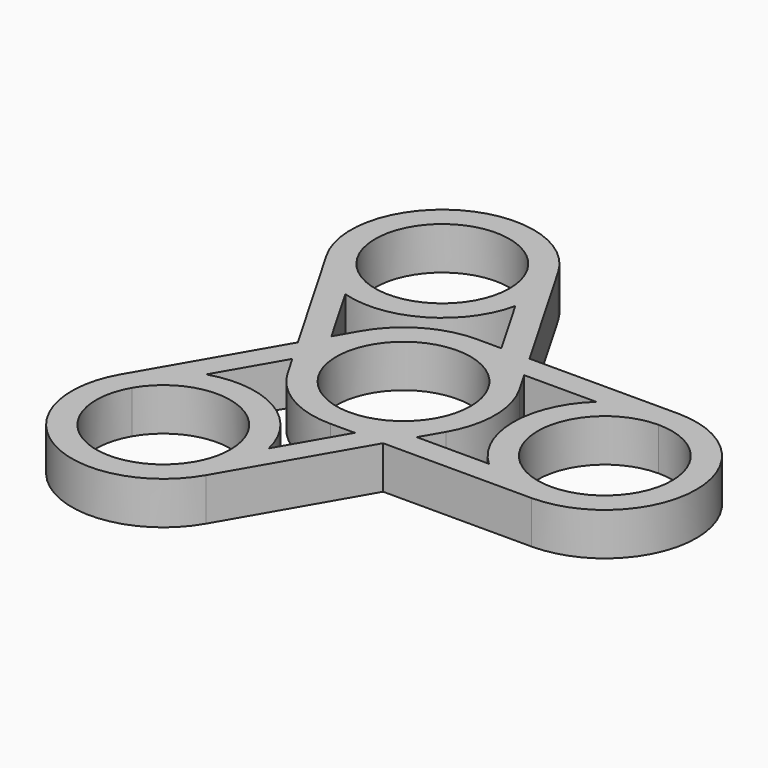
from build123d import *

# Parameters (mm, degrees)
F0_R     = 11
F1_DEPTH = 7


# Not quite as in the source:
# - a feature names something its author has since deleted; it is built from what else it names


with BuildPart() as f1:
    # F0 (on Top) → F1 (new body)
    with BuildSketch(Plane.XY):
        with BuildLine():
            Line((-15.0111069989, -4), (-12.9903810568, -7.5))
            ThreePointArc((-12.9903810568, -7.5), (-7.5, -12.9903810568), (0, -15))
            Line((0, -15), (4.0414518843, -15))
            Line((4.0414518843, -15), (-1.8747010448, -25.2470774586))
            ThreePointArc((-1.8747010448, -25.2470774586), (-1.5939696041, -26.9024559592), (-1.5, -28.5788383249))
            ThreePointArc((-1.5, -28.5788383249), (-2.0111126057, -32.4611240014), (-3.5096189432, -36.0788383249))
            Line((-3.5096189432, -36.0788383249), (8.6602540378, -15))
            Line((8.6602540378, -15), (33, -15))
            ThreePointArc((33, -15), (27.5227744249, -13.9642400438), (22.8019609728, -11))
            Line((22.8019609728, -11), (10.9696551146, -11))
            Line((10.9696551146, -11), (12.9903810568, -7.5))
            ThreePointArc((12.9903810568, -7.5), (15, 0), (12.9903810568, 7.5))
            Line((12.9903810568, 7.5), (10.9696551146, 11))
            Line((10.9696551146, 11), (22.8019609728, 11))
            ThreePointArc((22.8019609728, 11), (27.5227744249, 13.9642400438), (33, 15))
            Line((33, 15), (8.6602540378, 15))
            Line((8.6602540378, 15), (-3.5096189432, 36.0788383249))
            ThreePointArc((-3.5096189432, 36.0788383249), (-2.0111126057, 32.4611240014), (-1.5, 28.5788383249))
            ThreePointArc((-1.5, 28.5788383249), (-1.5939696041, 26.9024559592), (-1.8747010448, 25.2470774586))
            Line((-1.8747010448, 25.2470774586), (4.0414518843, 15))
            Line((4.0414518843, 15), (0, 15))
            ThreePointArc((0, 15), (-7.5, 12.9903810568), (-12.9903810568, 7.5))
            Line((-12.9903810568, 7.5), (-15.0111069989, 4))
            Line((-15.0111069989, 4), (-20.927259928, 14.2470774586))
            ThreePointArc((-20.927259928, 14.2470774586), (-25.8547738349, 16.8533018127), (-29.4903810568, 21.0788383249))
            Line((-29.4903810568, 21.0788383249), (-17.3205080757, 0))
            Line((-17.3205080757, 0), (-29.4903810568, -21.0788383249))
            ThreePointArc((-29.4903810568, -21.0788383249), (-25.8547738349, -16.8533018127), (-20.927259928, -14.2470774586))
            Line((-20.927259928, -14.2470774586), (-15.0111069989, -4))
        make_face()
        Circle(F0_R, mode=Mode.SUBTRACT)
        with BuildLine():
            Line((-26.0262794416, -23.0788383249), (-20.927259928, -14.2470774586))
            ThreePointArc((-20.927259928, -14.2470774586), (-25.8547738349, -16.8533018127), (-29.4903810568, -21.0788383249))
            ThreePointArc((-29.4903810568, -21.0788383249), (-24, -41.5692193817), (-3.5096189432, -36.0788383249))
            ThreePointArc((-3.5096189432, -36.0788383249), (-2.0111126057, -32.4611240014), (-1.5, -28.5788383249))
            ThreePointArc((-1.5, -28.5788383249), (-1.5939696041, -26.9024559592), (-1.8747010448, -25.2470774586))
            Line((-1.8747010448, -25.2470774586), (-6.9737205584, -34.0788383249))
            ThreePointArc((-6.9737205584, -34.0788383249), (-22, -38.1051177665), (-26.0262794416, -23.0788383249))
        make_face()
        with BuildLine():
            ThreePointArc((-3.5096189432, 36.0788383249), (-24, 41.5692193817), (-29.4903810568, 21.0788383249))
            ThreePointArc((-29.4903810568, 21.0788383249), (-25.8547738349, 16.8533018127), (-20.927259928, 14.2470774586))
            Line((-20.927259928, 14.2470774586), (-26.0262794416, 23.0788383249))
            ThreePointArc((-26.0262794416, 23.0788383249), (-22, 38.1051177665), (-6.9737205584, 34.0788383249))
            Line((-6.9737205584, 34.0788383249), (-1.8747010448, 25.2470774586))
            ThreePointArc((-1.8747010448, 25.2470774586), (-1.5939696041, 26.9024559592), (-1.5, 28.5788383249))
            ThreePointArc((-1.5, 28.5788383249), (-2.0111126057, 32.4611240014), (-3.5096189432, 36.0788383249))
        make_face()
        with BuildLine():
            ThreePointArc((22.8019609728, -11), (27.5227744249, -13.9642400438), (33, -15))
            ThreePointArc((33, -15), (43.6066017178, -10.6066017178), (48, 0))
            ThreePointArc((48, 0), (43.6066017178, 10.6066017178), (33, 15))
            ThreePointArc((33, 15), (27.5227744249, 13.9642400438), (22.8019609728, 11))
            Line((22.8019609728, 11), (33, 11))
            ThreePointArc((33, 11), (40.7781745931, 7.7781745931), (44, 0))
            ThreePointArc((44, 0), (40.7781745931, -7.7781745931), (33, -11))
            Line((33, -11), (22.8019609728, -11))
        make_face()
        with BuildLine():
            ThreePointArc((22.8019609728, 11), (18, 0), (22.8019609728, -11))
            Line((22.8019609728, -11), (33, -11))
            ThreePointArc((33, -11), (22, 0), (33, 11))
            Line((33, 11), (22.8019609728, 11))
        make_face()
        with BuildLine():
            Line((-26.0262794416, 23.0788383249), (-20.927259928, 14.2470774586))
            ThreePointArc((-20.927259928, 14.2470774586), (-9, 15.5884572681), (-1.8747010448, 25.2470774586))
            Line((-1.8747010448, 25.2470774586), (-6.9737205584, 34.0788383249))
            ThreePointArc((-6.9737205584, 34.0788383249), (-5.8748159108, 31.425847821), (-5.5, 28.5788383249))
            ThreePointArc((-5.5, 28.5788383249), (-13.6529905039, 17.9536542357), (-26.0262794416, 23.0788383249))
        make_face()
        with BuildLine():
            ThreePointArc((-1.8747010448, -25.2470774586), (-9, -15.5884572681), (-20.927259928, -14.2470774586))
            Line((-20.927259928, -14.2470774586), (-26.0262794416, -23.0788383249))
            ThreePointArc((-26.0262794416, -23.0788383249), (-13.6529905039, -17.9536542357), (-5.5, -28.5788383249))
            ThreePointArc((-5.5, -28.5788383249), (-5.8748159108, -31.425847821), (-6.9737205584, -34.0788383249))
            Line((-6.9737205584, -34.0788383249), (-1.8747010448, -25.2470774586))
        make_face()
    extrude(amount=F1_DEPTH)


solid = f1.part
